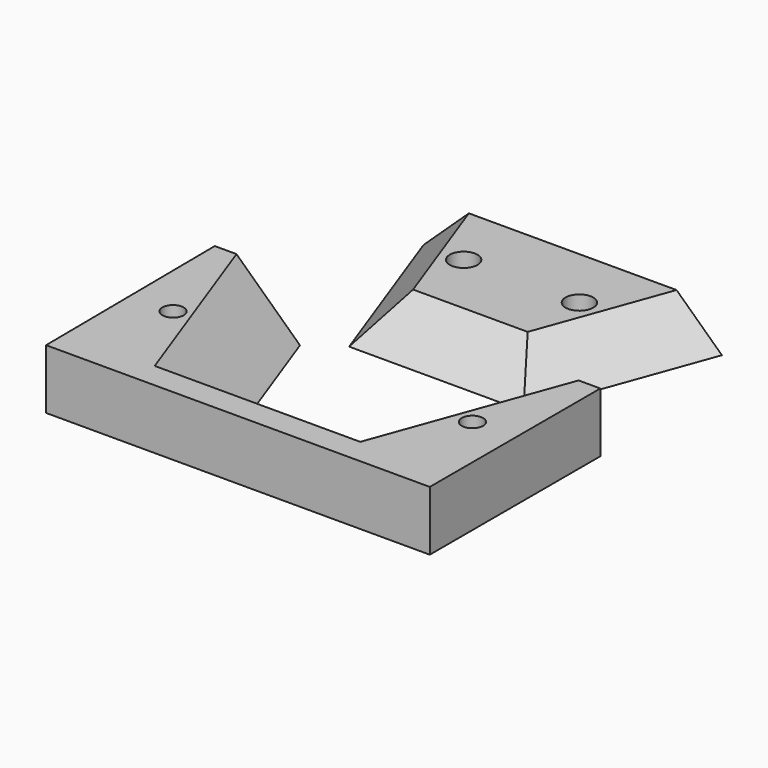
from build123d import *

# Parameters (mm, degrees)
F0_R           = 2.5
F1_DEPTH       = 14
F2_SIZE        = 13.99999
F3_R           = 3.25
F4_DEPTH       = 10
F5_SIZE        = 9.99999
F6_D           = 6.5
F6_CBORE_D     = 12
F6_CBORE_DEPTH = 5
F7_D           = 6.5
F7_CBORE_D     = 12
F7_CBORE_DEPTH = 5
F8_D           = 5
F8_CBORE_D     = 8.5
F8_CBORE_DEPTH = 3
F9_D           = 5
F9_CBORE_D     = 8.5
F9_CBORE_DEPTH = 3


# Not quite as in the source:
# - a fillet or chamfer is up to 0.001 mm smaller than in the source, because OpenCascade refuses the exact size


with BuildPart() as f1:
    # F0 (on Top) → F1 (new body)
    with BuildSketch(Plane.XY):
        Polygon((-19.0606748313, 23.7515140325), (-39.0606748313, 23.7515140325), (-38.6201621495, -26.2465454156), (51.3798378505, -26.2465454156), (51.3798378505, 23.7534545844), (31.3798378505, 23.7534545844), (20.4607308225, -6.2465454156), (-8.1422741064, -6.2465454156), align=None)
        with Locations((-28.8400389136, -1.2465454156)):
            Circle(F0_R, mode=Mode.SUBTRACT)
        with Locations((41.3798378505, -1.2465454156)):
            Circle(F0_R, mode=Mode.SUBTRACT)
    extrude(amount=F1_DEPTH)

    # F2 (size 14 in the source; OpenCascade refuses exactly that, so slightly less here)
    f2_edges = [f1.edges().sort_by_distance(p)[0] for p in [
        (-13.601474, 8.752484, 14),
        (6.159228, -6.246545, 14),
        (25.920284, 8.753455, 14),
    ]]
    chamfer(f2_edges, length=F2_SIZE)

    # F8 (through all)
    with Locations(Plane(origin=(0, 0, 0), x_dir=(1, 0, 0), z_dir=(0, 0, -1))):
        with Locations((-28.8400389136, 1.2465454156)):
            CounterBoreHole(F8_D / 2, F8_CBORE_D / 2, F8_CBORE_DEPTH)

    # F9 (through all)
    with Locations(Plane(origin=(0, 0, 0), x_dir=(1, 0, 0), z_dir=(0, 0, -1))):
        with Locations((41.3798378505, 1.2465454156)):
            CounterBoreHole(F9_D / 2, F9_CBORE_D / 2, F9_CBORE_DEPTH)


with BuildPart() as f4:
    # F3 (on Top) → F4 (new body)
    with BuildSketch(Plane.XY):
        Polygon((43.7290843949, 68.9680808707), (-26.2709156051, 68.9680808707), (-11.7121062345, 28.9680808707), (29.1702750242, 28.9680808707), align=None)
        with Locations((-4.848695504, 53.9680808707)):
            Circle(F3_R, mode=Mode.SUBTRACT)
        with Locations((22.3068642937, 53.9680808707)):
            Circle(F3_R, mode=Mode.SUBTRACT)
    extrude(amount=F4_DEPTH)

    # F5 (size 10 in the source; OpenCascade refuses exactly that, so slightly less here)
    f5_edges = [f4.edges().sort_by_distance(p)[0] for p in [
        (8.729084, 28.968081, 10),
        (-18.991511, 48.968081, 10),
        (36.44968, 48.968081, 10),
    ]]
    chamfer(f5_edges, length=F5_SIZE)

    # F6 (through all)
    with Locations(Plane(origin=(0, 0, 0), x_dir=(1, 0, 0), z_dir=(0, 0, -1))):
        with Locations((-4.848695504, -53.9680808707)):
            CounterBoreHole(F6_D / 2, F6_CBORE_D / 2, F6_CBORE_DEPTH)

    # F7 (through all)
    with Locations(Plane(origin=(0, 0, 0), x_dir=(1, 0, 0), z_dir=(0, 0, -1))):
        with Locations((22.3068642937, -53.9680808707)):
            CounterBoreHole(F7_D / 2, F7_CBORE_D / 2, F7_CBORE_DEPTH)


solid = Compound([f1.part, f4.part])
